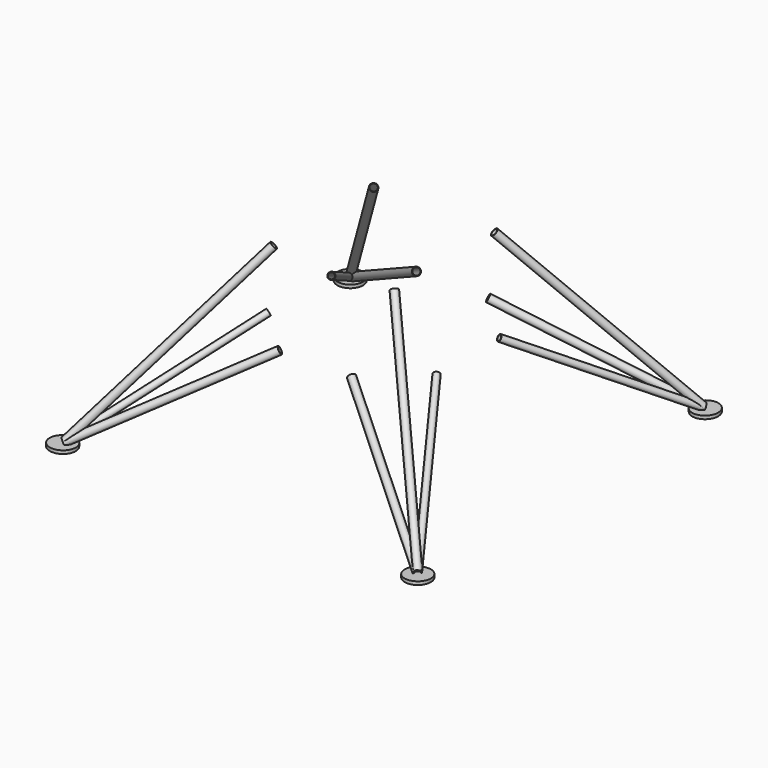
from build123d import *
from build123d import SkipClean  # not in build123d's __all__

# Parameters (mm, degrees)
F11_R     = 300
F12_DEPTH = 75


with BuildPart() as f6:
    # F5 (on face) → F6 (revolve)
    with BuildSketch(Plane(origin=(972.3486103798, -972.3486103798, 2575.3495425425), x_dir=(0.9429071555, 0.1176426496, -0.3115867505), z_dir=(-0.3330556952, 0.3330556952, -0.882126866))):
        Polygon((3246.0507254627, 3836.9942274935), (964.8005575818, 98.4438953418), (975.044106126, 92.1933183106), (3256.2942740069, 3830.7436504624), align=None)
    revolve(axis=Axis((3010.9069657282, -2510.9069657282, 1224.7738613173), (-0.4911428174, 0.7373257993, 0.4638204378)))

    # F7 (on face) → F8 (revolve)
    with BuildSketch(Plane(origin=(972.3486103798, -972.3486103798, 2575.3495425425), x_dir=(0.9429071555, 0.1176426496, -0.3115867505), z_dir=(-0.3330556952, 0.3330556952, -0.882126866))):
        Polygon((-205.4840400391, 1120.0597335932), (-198.0042582697, 1110.6760847995), (3255.4915883993, 3863.4853429461), (3248.0118066299, 3872.8689917398), align=None)
    with SkipClean():  # cleaning this boolean's faces spoils the solid; the shape is the same uncleaned
        revolve(axis=Axis((2460.9069657282, -3060.9069657282, 1224.7738613173), (-0.7373257993, 0.4911428174, 0.4638204378)))

    # F11 (on face) → F12 (join)
    with BuildSketch(Plane(origin=(-1.055572279, 1.055572279, 106.9073084662), x_dir=(0.9999512632, 9.7476e-05, 0.0098722712), z_dir=(-0.0098727524, 0.0098727524, 0.999902524))):
        with Locations((4109.4301739364, -4159.8332209603)):
            Circle(F11_R)
    with SkipClean():  # cleaning this boolean's faces spoils the solid; the shape is the same uncleaned
        extrude(amount=-F12_DEPTH)

    # F14 (on face) → F15 (revolve)
    with BuildSketch(Plane(origin=(-25, -25, 0), x_dir=(-0.7071067812, 0.7071067812, 0), z_dir=(0.7071067812, 0.7071067812, 0))):
        Polygon((-1948.474921207, 3928.6372845481), (-1956.9228000959, 3937.1598042623), (-5756.8814387573, 170.4814697917), (-5748.4335598684, 161.9589500776), align=None)
    with SkipClean():  # cleaning this boolean's faces spoils the solid; the shape is the same uncleaned
        revolve(axis=Axis((2727.0214885701, -2777.0214885701, 2124.6861329257), (0.5021942902, -0.5021942902, -0.7039899074)))


with BuildPart() as f16_1:
    # F16: instance of F6
    add(f6.part.mirror(Plane.XZ), clean=False)


with BuildPart() as f17_1:
    # F17: instance of F6
    add(f6.part.mirror(Plane.YZ), clean=False)


with BuildPart() as f17_2:
    # F17: instance of F16_1
    add(f16_1.part.mirror(Plane.YZ), clean=False)


solid = Compound([f6.part, f16_1.part, f17_1.part, f17_2.part])
